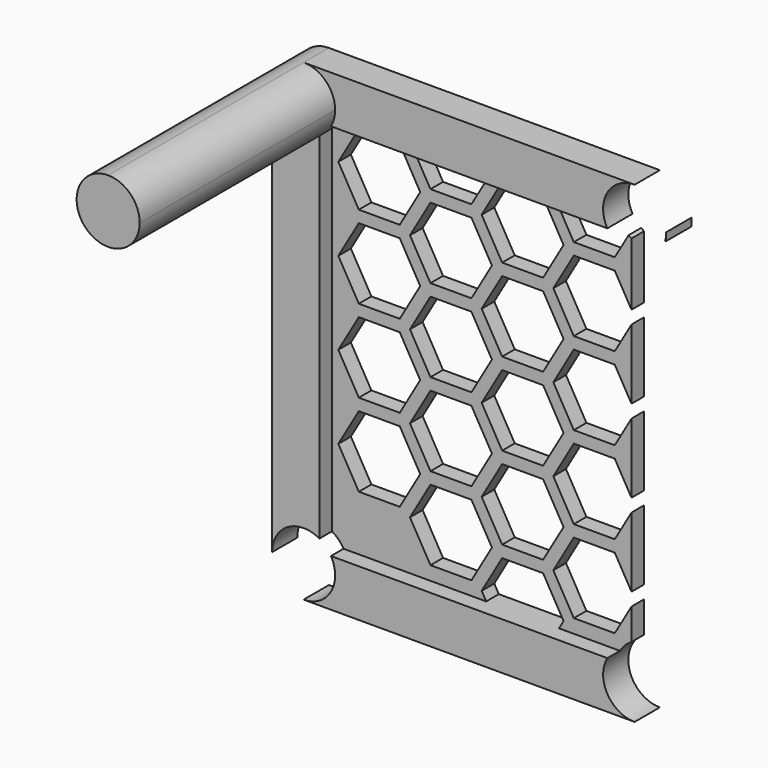
from build123d import *

# Parameters (mm, degrees)
F1_DEPTH = 2
F2_DEPTH = 4
F3_DEPTH = 35


# Not quite as in the source:
# - a feature of the source that left no trace in its solid (it failed there, or was rolled back) is left out
# - a feature names something its author has since deleted; it is built from what else it names


with BuildPart() as f1:
    # F0 (on Front) → F1 (new body)
    with BuildSketch(Plane.XZ):
        with BuildLine():
            Line((-8.9585481157, 24), (-17.5358983849, 24))
            ThreePointArc((-17.5358983849, 24), (-18.1715728753, 23.1715728753), (-19, 22.5358983849))
            Line((-19, 22.5358983849), (-19, -22.5358983849))
            ThreePointArc((-19, -22.5358983849), (-18.1715728753, -23.1715728753), (-17.5358983849, -24))
            Line((-17.5358983849, -24), (-8.3811978465, -24))
            Line((-8.3811978465, -24), (0.567731326, -24))
            Line((0.567731326, -24), (-0.0096189432, -23))
            Line((-0.0096189432, -23), (2.5884572681, -18.5))
            Line((2.5884572681, -18.5), (7.7846096908, -18.5))
            Line((7.7846096908, -18.5), (10.3826859022, -23))
            Line((10.3826859022, -23), (9.805335633, -24))
            Line((9.805335633, -24), (17.5358983849, -24))
            ThreePointArc((17.5358983849, -24), (18.1715728753, -23.1715728753), (19, -22.5358983849))
            Line((19, -22.5358983849), (19, -18.5743741578))
            Line((19, -18.5743741578), (16.8778764306, -22.25))
            Line((16.8778764306, -22.25), (11.6817240079, -22.25))
            Line((11.6817240079, -22.25), (9.0836477965, -17.75))
            Line((9.0836477965, -17.75), (11.6817240079, -13.25))
            Line((11.6817240079, -13.25), (16.8778764306, -13.25))
            Line((16.8778764306, -13.25), (19, -16.9256258422))
            Line((19, -16.9256258422), (19, -8.0743741578))
            Line((19, -8.0743741578), (16.8778764306, -11.75))
            Line((16.8778764306, -11.75), (11.6817240079, -11.75))
            Line((11.6817240079, -11.75), (9.0836477965, -7.25))
            Line((9.0836477965, -7.25), (11.6817240079, -2.75))
            Line((11.6817240079, -2.75), (16.8778764306, -2.75))
            Line((16.8778764306, -2.75), (19, -6.4256258422))
            Line((19, -6.4256258422), (19, 2.4256258422))
            Line((19, 2.4256258422), (16.8778764306, -1.25))
            Line((16.8778764306, -1.25), (11.6817240079, -1.25))
            Line((11.6817240079, -1.25), (9.0836477965, 3.25))
            Line((9.0836477965, 3.25), (11.6817240079, 7.75))
            Line((11.6817240079, 7.75), (16.8778764306, 7.75))
            Line((16.8778764306, 7.75), (19, 4.0743741578))
            Line((19, 4.0743741578), (19, 12.9256258422))
            Line((19, 12.9256258422), (16.8778764306, 9.25))
            Line((16.8778764306, 9.25), (11.6817240079, 9.25))
            Line((11.6817240079, 9.25), (9.0836477965, 13.75))
            Line((9.0836477965, 13.75), (11.6817240079, 18.25))
            Line((11.6817240079, 18.25), (16.8778764306, 18.25))
            Line((16.8778764306, 18.25), (19, 14.5743741578))
            Line((19, 14.5743741578), (19, 22.5358983849))
            ThreePointArc((19, 22.5358983849), (18.8101731757, 22.6526639727), (18.6271441796, 22.7798206174))
            Line((18.6271441796, 22.7798206174), (16.8778764306, 19.75))
            Line((16.8778764306, 19.75), (11.6817240079, 19.75))
            Line((11.6817240079, 19.75), (9.2279853638, 24))
            Line((9.2279853638, 24), (1.1450815951, 24))
            Line((1.1450815951, 24), (-1.3086570489, 19.75))
            Line((-1.3086570489, 19.75), (-6.5048094716, 19.75))
            Line((-6.5048094716, 19.75), (-8.9585481157, 24))
        make_face()
        Polygon((1.2894191624, -17.75), (-1.3086570489, -22.25), (-6.5048094716, -22.25), (-9.102885683, -17.75), (-6.5048094716, -13.25), (-1.3086570489, -13.25), align=None, mode=Mode.SUBTRACT)
        Polygon((-7.8038475773, -12.5), (-10.4019237886, -17), (-15.5980762114, -17), (-18.1961524227, -12.5), (-15.5980762114, -8), (-10.4019237886, -8), align=None, mode=Mode.SUBTRACT)
        Polygon((-7.8038475773, -2), (-10.4019237886, -6.5), (-15.5980762114, -6.5), (-18.1961524227, -2), (-15.5980762114, 2.5), (-10.4019237886, 2.5), align=None, mode=Mode.SUBTRACT)
        Polygon((1.2894191624, -7.25), (-1.3086570489, -11.75), (-6.5048094716, -11.75), (-9.102885683, -7.25), (-6.5048094716, -2.75), (-1.3086570489, -2.75), align=None, mode=Mode.SUBTRACT)
        Polygon((10.3826859022, -12.5), (7.7846096908, -17), (2.5884572681, -17), (-0.0096189432, -12.5), (2.5884572681, -8), (7.7846096908, -8), align=None, mode=Mode.SUBTRACT)
        Polygon((10.3826859022, -2), (7.7846096908, -6.5), (2.5884572681, -6.5), (-0.0096189432, -2), (2.5884572681, 2.5), (7.7846096908, 2.5), align=None, mode=Mode.SUBTRACT)
        Polygon((-7.8038475773, 8.5), (-10.4019237886, 4), (-15.5980762114, 4), (-18.1961524227, 8.5), (-15.5980762114, 13), (-10.4019237886, 13), align=None, mode=Mode.SUBTRACT)
        Polygon((1.2894191624, 3.25), (-1.3086570489, -1.25), (-6.5048094716, -1.25), (-9.102885683, 3.25), (-6.5048094716, 7.75), (-1.3086570489, 7.75), align=None, mode=Mode.SUBTRACT)
        Polygon((1.2894191624, 13.75), (-1.3086570489, 9.25), (-6.5048094716, 9.25), (-9.102885683, 13.75), (-6.5048094716, 18.25), (-1.3086570489, 18.25), align=None, mode=Mode.SUBTRACT)
        Polygon((-10.4019237886, 23.5), (-7.8038475773, 19), (-10.4019237886, 14.5), (-15.5980762114, 14.5), (-18.1961524227, 19), (-15.5980762114, 23.5), align=None, mode=Mode.SUBTRACT)
        Polygon((10.3826859022, 8.5), (7.7846096908, 4), (2.5884572681, 4), (-0.0096189432, 8.5), (2.5884572681, 13), (7.7846096908, 13), align=None, mode=Mode.SUBTRACT)
        Polygon((10.3826859022, 19), (7.7846096908, 14.5), (2.5884572681, 14.5), (-0.0096189432, 19), (2.5884572681, 23.5), (7.7846096908, 23.5), align=None, mode=Mode.SUBTRACT)
    extrude(amount=F1_DEPTH)

    # F0 (on Front) → F2, piece 2 (join)
    with BuildSketch(Plane.XZ):
        with BuildLine():
            Line((21, 30), (-21, 30))
            ThreePointArc((-21, 30), (-18.1715728753, 28.8284271247), (-17, 26))
            ThreePointArc((-17, 26), (-17.1362966948, 24.9647238196), (-17.5358983849, 24))
            Line((-17.5358983849, 24), (-8.9585481157, 24))
            Line((-8.9585481157, 24), (1.1450815951, 24))
            Line((1.1450815951, 24), (9.2279853638, 24))
            Line((9.2279853638, 24), (17.5358983849, 24))
            ThreePointArc((17.5358983849, 24), (17.5358983849, 28), (21, 30))
        make_face()
        with BuildLine():
            ThreePointArc((-19, 22.5358983849), (-23, 22.5358983849), (-25, 26))
            Line((-25, 26), (-25, -26))
            ThreePointArc((-25, -26), (-23, -22.5358983849), (-19, -22.5358983849))
            Line((-19, -22.5358983849), (-19, 22.5358983849))
        make_face()
        with BuildLine():
            ThreePointArc((-17, -26), (-18.1715728753, -28.8284271247), (-21, -30))
            Line((-21, -30), (21, -30))
            ThreePointArc((21, -30), (17.5358983849, -28), (17.5358983849, -24))
            Line((17.5358983849, -24), (9.805335633, -24))
            Line((9.805335633, -24), (0.567731326, -24))
            Line((0.567731326, -24), (-8.3811978465, -24))
            Line((-8.3811978465, -24), (-17.5358983849, -24))
            ThreePointArc((-17.5358983849, -24), (-17.1362966948, -24.9647238196), (-17, -26))
        make_face()
    extrude(amount=F2_DEPTH)

    # F0 (on Front) → F3 (join)
    with BuildSketch(Plane.XZ):
        with BuildLine():
            ThreePointArc((-17, 26), (-18.1715728753, 28.8284271247), (-21, 30))
            ThreePointArc((-21, 30), (-23.8284271247, 28.8284271247), (-25, 26))
            ThreePointArc((-25, 26), (-23, 22.5358983849), (-19, 22.5358983849))
            ThreePointArc((-19, 22.5358983849), (-18.1715728753, 23.1715728753), (-17.5358983849, 24))
            ThreePointArc((-17.5358983849, 24), (-17.1362966948, 24.9647238196), (-17, 26))
        make_face()
    extrude(amount=F3_DEPTH)


with BuildPart() as f2:
    # F0 (on Front) → F2 (new body)
    with BuildSketch(Plane.XZ):
        with BuildLine():
            Line((25, 25), (25, 26))
            ThreePointArc((25, 26), (24.9681187851, 25.4959828301), (24.8729833462, 25))
            Line((24.8729833462, 25), (25, 25))
        make_face()
    extrude(amount=F2_DEPTH)


solid = Compound([f1.part, f2.part])
